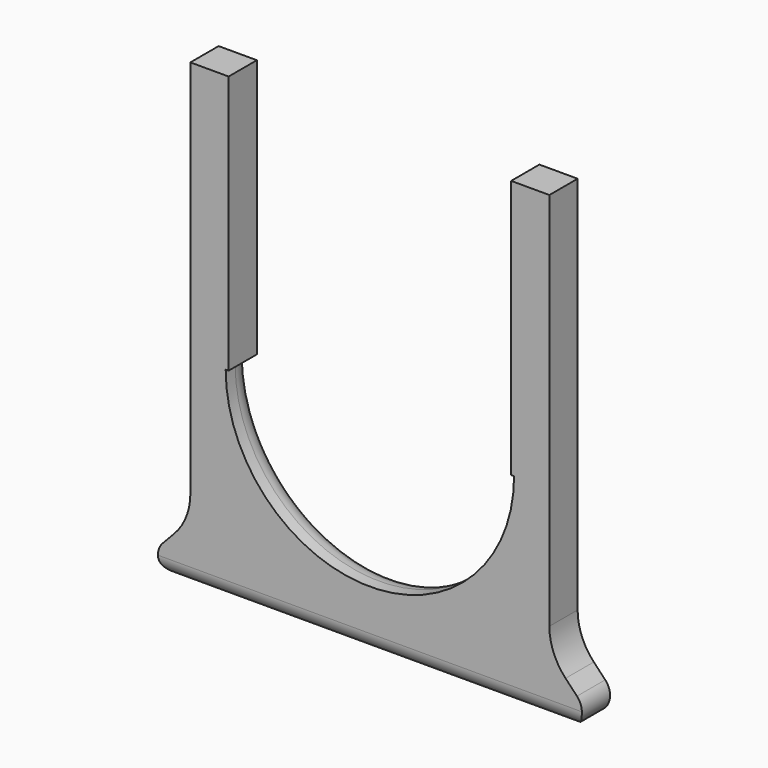
from build123d import *

# Parameters (mm, degrees)
F1_DEPTH    = 3
F2_DEPTH    = 0.25
F3_DEPTH    = 0.25
F4_R        = 2
F5_R        = 1.5
F6_R        = 5
F7_T1_DEPTH = 40.5120657328


# Not quite as in the source:
# - a fillet or chamfer that OpenCascade refuses, or shapes differently, is made with other operations: its cross-section is extruded or revolved along the edge and cut away or added


with BuildPart() as f1:
    # F0 (on Front) → F1 (new body)
    with BuildSketch(Plane.XZ):
        with BuildLine():
            ThreePointArc((3.6544098407, -9.5319570974), (-8.5955901593, -21.7819570974), (-20.8455901593, -9.5319570974))
            Line((-20.8455901593, -9.5319570974), (-20.8455901593, 12.4680429026))
            Line((-20.8455901593, 12.4680429026), (-23.8455901593, 12.4680429026))
            Line((-23.8455901593, 12.4680429026), (-23.8455901593, -9.5319570974))
            Line((-23.8455901593, -9.5319570974), (-23.8455901593, -21.7819570974))
            Line((-23.8455901593, -21.7819570974), (-28.5955901593, -26.7819570974))
            Line((-28.5955901593, -26.7819570974), (-8.5955901593, -26.7819570974))
            Line((-8.5955901593, -26.7819570974), (11.4044098407, -26.7819570974))
            Line((11.4044098407, -26.7819570974), (6.6544098407, -21.7819570974))
            Line((6.6544098407, -21.7819570974), (6.6544098407, 12.4680429026))
            Line((6.6544098407, 12.4680429026), (3.6544098407, 12.4680429026))
            Line((3.6544098407, 12.4680429026), (3.6544098407, -9.5319570974))
        make_face()
    extrude(amount=F1_DEPTH)

    # F2 (add): a face of the model
    f2_faces = [f1.faces().sort_by_distance(p)[0] for p in [
        (-20.8455901593, -1.5, 1.4680429026),
    ]]
    extrude(f2_faces, amount=F2_DEPTH)

    # F3 (add): a face of the model
    f3_faces = [f1.faces().sort_by_distance(p)[0] for p in [
        (3.6544098407, -1.5, 1.4680429026),
    ]]
    extrude(f3_faces, amount=F3_DEPTH)

    # F4
    f4_edges = [f1.edges().sort_by_distance(p)[0] for p in [
        (-8.59559, 0, -21.781957),
    ]]
    fillet(f4_edges, radius=F4_R)

    # F5
    f5_edges = [f1.edges().sort_by_distance(p)[0] for p in [
        (11.40441, -1.5, -26.781957),
        (-28.59559, -1.5, -26.781957),
    ]]
    fillet(f5_edges, radius=F5_R)

    # F6
    f6_edges = [f1.edges().sort_by_distance(p)[0] for p in [
        (-23.84559, -1.5, -21.781957),
        (6.65441, -1.5, -21.781957),
    ]]
    fillet(f6_edges, radius=F6_R)

    # F7: fillet of radius 1.5 on 1 edges, made by hand

    # F7_s2 → F7_t1 (cut)
    with BuildSketch(Plane.YZ.offset(-28.8516230257)):
        with BuildLine():
            ThreePointArc((-3, -25.2819570974), (-2.5606601718, -26.3426172691), (-1.5, -26.7819570974))
            Line((-1.5, -26.7819570974), (-3, -26.7819570974))
            Line((-3, -26.7819570974), (-3, -25.2819570974))
        make_face()
    extrude(amount=F7_T1_DEPTH, mode=Mode.SUBTRACT)


solid = f1.part
